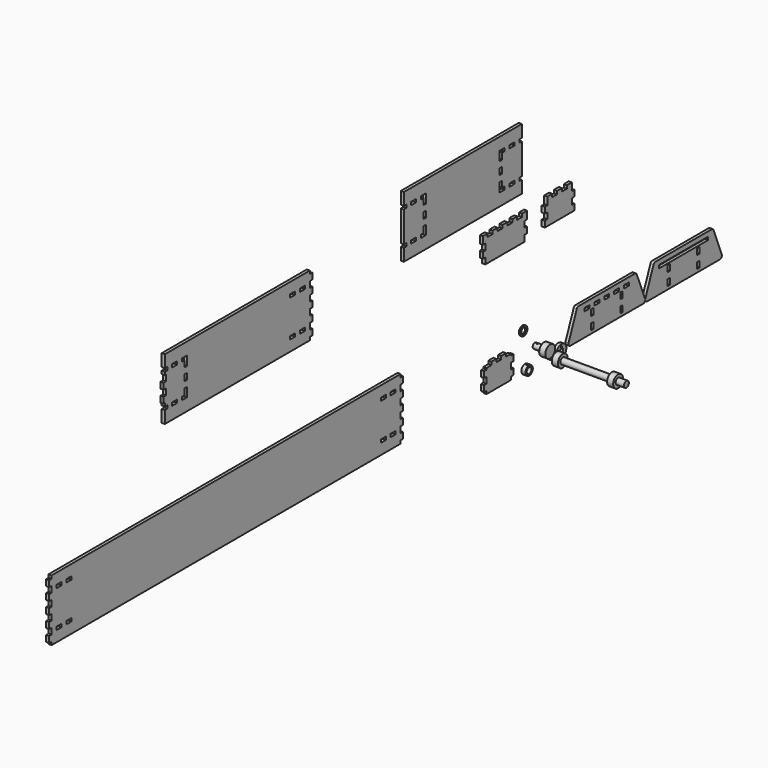
from build123d import *

# Parameters (mm, degrees)
F0_W      = 152.4
F0_H      = 101.6
F0_W_2    = 6.35
F0_H_2    = 12.7
F1_DEPTH  = 6.35
F2_W      = 152.4
F2_H      = 101.6
F2_W_2    = 6.35
F2_H_2    = 12.7
F2_W_3    = 127
F2_H_3    = 6.35
F3_DEPTH  = 6.35
F5_DEPTH  = 6.35
F6_W      = 12.7
F6_H      = 6.35
F7_DEPTH  = 6.35
F8_R      = 5.715
F9_DEPTH  = 19.05
F10_R     = 5.715
F11_DEPTH = 17.145
F12_R     = 12.7
F12_R_2   = 5.715
F13_DEPTH = 12.7
F14_R     = 6.35
F15_DEPTH = 101.6
F16_R     = 12.7
F16_R_2   = 6.35
F17_DEPTH = 12.7
F18_R     = 6.35
F19_DEPTH = 17.145
F20_R     = 12.7
F20_R_2   = 5.715
F21_DEPTH = 12.7
F22_R     = 1.5875
F23_DEPTH = 127.001
F24_R     = 9.525
F25_DEPTH = 8.4666666667
F26_R     = 1.5875
F27_DEPTH = 127.001
F28_R     = 6.35
F29_DEPTH = 8.4676667667
F30_R     = 9.525
F30_R_2   = 6.35
F31_DEPTH = 2.38125
F35_DEPTH = 6.35
F37_DEPTH = 6.35
F38_W     = 12.7
F38_H     = 6.35
F38_W_2   = 6.35
F38_H_2   = 12.7
F39_DEPTH = 6.35
F40_W     = 12.7
F40_H     = 6.35
F40_W_2   = 3.175
F40_H_2   = 12.7
F41_DEPTH = 6.35
F42_W     = 152.4
F42_H     = 38.1
F43_DEPTH = 6.35
F44_W     = 152.4
F44_H     = 38.1
F45_DEPTH = 6.35
F47_DEPTH = 6.35
F48_R     = 5.08
F50_DEPTH = 6.35
F51_R     = 5.08
F52_R     = 12.7
F52_R_2   = 1.524
F52_R_3   = 4.445
F53_DEPTH = 6.35


with BuildPart() as f1:
    # F0 (on Right) → F1 (new body)
    with BuildSketch(Plane.YZ):
        with Locations((76.2, 50.8)):
            Rectangle(F0_W, F0_H)
        with Locations((38.1, 12.7)):
            Rectangle(F0_W_2, F0_H_2, mode=Mode.SUBTRACT)
        with Locations((38.1, 38.1)):
            Rectangle(F0_W_2, F0_H_2, mode=Mode.SUBTRACT)
        Polygon((19.05, 53.975), (25.4, 53.975), (31.75, 53.975), (31.75, 50.8), (31.75, 47.625), (25.4, 47.625), (19.05, 47.625), (19.05, 50.8), align=None, mode=Mode.SUBTRACT)
        Polygon((44.45, 53.975), (50.8, 53.975), (57.15, 53.975), (57.15, 50.8), (57.15, 47.625), (50.8, 47.625), (44.45, 47.625), (44.45, 50.8), align=None, mode=Mode.SUBTRACT)
        Polygon((69.85, 53.975), (76.2, 53.975), (82.55, 53.975), (82.55, 50.8), (82.55, 47.625), (76.2, 47.625), (69.85, 47.625), (69.85, 50.8), align=None, mode=Mode.SUBTRACT)
        with Locations((114.3, 12.7)):
            Rectangle(F0_W_2, F0_H_2, mode=Mode.SUBTRACT)
        Polygon((95.25, 53.975), (101.6, 53.975), (107.95, 53.975), (107.95, 50.8), (107.95, 47.625), (101.6, 47.625), (95.25, 47.625), (95.25, 50.8), align=None, mode=Mode.SUBTRACT)
        with Locations((114.3, 38.1)):
            Rectangle(F0_W_2, F0_H_2, mode=Mode.SUBTRACT)
        Polygon((120.65, 53.975), (127, 53.975), (133.35, 53.975), (133.35, 50.8), (133.35, 47.625), (127, 47.625), (120.65, 47.625), (120.65, 50.8), align=None, mode=Mode.SUBTRACT)
    extrude(amount=F1_DEPTH)

    # F44 (on face) → F45 (cut, through all)
    with BuildSketch(Plane(origin=(0, 0, 0), x_dir=(0, -1, 0), z_dir=(-1, 0, 0))):
        with Locations((-76.2, 82.55)):
            Rectangle(F44_W, F44_H)
    extrude(amount=-F45_DEPTH, mode=Mode.SUBTRACT)

    # F49 (on face) → F50 (join)
    with BuildSketch(Plane(origin=(0, 0, 0), x_dir=(0, -1, 0), z_dir=(-1, 0, 0))):
        Polygon((-152.4, 0), (-152.4, 63.5), (-177.8, 0), align=None)
        Polygon((25.4, 0), (0, 63.5), (0, 0), align=None)
    extrude(amount=-F50_DEPTH)

    # F51
    f51_edges = [f1.edges().sort_by_distance(p)[0] for p in [
        (3.175, 152.4, 63.5),
        (3.175, 0, 63.5),
        (3.175, -25.4, 0),
        (3.175, 177.8, 0),
    ]]
    fillet(f51_edges, radius=F51_R)


with BuildPart() as f3:
    # F2 (on Right) → F3 (new body)
    with BuildSketch(Plane.YZ):
        with Locations((274.5815088749, 50.8)):
            Rectangle(F2_W, F2_H)
        with Locations((236.4815088749, 12.7)):
            Rectangle(F2_W_2, F2_H_2, mode=Mode.SUBTRACT)
        with Locations((236.4815088749, 38.1)):
            Rectangle(F2_W_2, F2_H_2, mode=Mode.SUBTRACT)
        with Locations((274.5815088749, 50.8)):
            Rectangle(F2_W_3, F2_H_3, mode=Mode.SUBTRACT)
        with Locations((312.6815088749, 12.7)):
            Rectangle(F2_W_2, F2_H_2, mode=Mode.SUBTRACT)
        with Locations((312.6815088749, 38.1)):
            Rectangle(F2_W_2, F2_H_2, mode=Mode.SUBTRACT)
    extrude(amount=F3_DEPTH)

    # F42 (on face) → F43 (cut, through all)
    with BuildSketch(Plane(origin=(0, 0, 0), x_dir=(0, -1, 0), z_dir=(-1, 0, 0))):
        with Locations((-274.5815088749, 82.55)):
            Rectangle(F42_W, F42_H)
    extrude(amount=-F43_DEPTH, mode=Mode.SUBTRACT)

    # F46 (on face) → F47 (join)
    with BuildSketch(Plane(origin=(0, 0, 0), x_dir=(0, -1, 0), z_dir=(-1, 0, 0))):
        Polygon((-350.7815088749, 0), (-350.7815088749, 63.5), (-376.1815088749, 0), align=None)
        Polygon((-172.9815088749, 0), (-198.3815088749, 63.5), (-198.3815088749, 0), align=None)
    extrude(amount=-F47_DEPTH)

    # F48
    f48_edges = [f3.edges().sort_by_distance(p)[0] for p in [
        (3.175, 350.781509, 63.5),
        (3.175, 198.381509, 63.5),
        (3.175, 376.181509, 0),
        (3.175, 172.981509, 0),
    ]]
    fillet(f48_edges, radius=F48_R)


with BuildPart() as f5:
    # F4 (on Right) → F5 (new body)
    with BuildSketch(Plane.YZ):
        Polygon((-234.6794404593, 0), (-171.1794404593, 0), (-171.1794404593, 6.35), (-164.8294404593, 6.35), (-164.8294404593, 19.05), (-171.1794404593, 19.05), (-171.1794404593, 31.75), (-164.8294404593, 31.75), (-164.8294404593, 44.45), (-171.1794404593, 44.45), (-171.1794404593, 47.625), (-183.8794404593, 47.625), (-183.8794404593, 53.975), (-196.5794404593, 53.975), (-196.5794404593, 47.625), (-202.9294404593, 47.625), (-209.2794404593, 47.625), (-209.2794404593, 53.975), (-221.9794404593, 53.975), (-221.9794404593, 47.625), (-234.6794404593, 47.625), (-234.6794404593, 44.45), (-241.0294404593, 44.45), (-241.0294404593, 31.75), (-234.6794404593, 31.75), (-234.6794404593, 19.05), (-241.0294404593, 19.05), (-241.0294404593, 6.35), (-234.6794404593, 6.35), align=None)
    extrude(amount=F5_DEPTH)


with BuildPart() as f7:
    # F6 (on Right) → F7 (new body)
    with BuildSketch(Plane.YZ):
        Polygon((-1358.3947817802, 0), (-456.6947817802, 0), (-456.6947817802, 6.35), (-450.3447817802, 6.35), (-450.3447817802, 19.05), (-456.6947817802, 19.05), (-456.6947817802, 22.225), (-456.6947817802, 28.575), (-456.6947817802, 31.75), (-450.3447817802, 31.75), (-450.3447817802, 44.45), (-456.6947817802, 44.45), (-456.6947817802, 57.15), (-450.3447817802, 57.15), (-450.3447817802, 69.85), (-456.6947817802, 69.85), (-456.6947817802, 82.55), (-450.3447817802, 82.55), (-450.3447817802, 95.25), (-456.6947817802, 95.25), (-456.6947817802, 98.425), (-456.6947817802, 104.775), (-456.6947817802, 107.95), (-450.3447817802, 107.95), (-450.3447817802, 120.65), (-456.6947817802, 120.65), (-456.6947817802, 127), (-1358.3947817802, 127), (-1358.3947817802, 120.65), (-1364.7447817802, 120.65), (-1364.7447817802, 107.95), (-1358.3947817802, 107.95), (-1358.3947817802, 104.775), (-1358.3947817802, 98.425), (-1358.3947817802, 95.25), (-1364.7447817802, 95.25), (-1364.7447817802, 82.55), (-1358.3947817802, 82.55), (-1358.3947817802, 69.85), (-1364.7447817802, 69.85), (-1364.7447817802, 57.15), (-1358.3947817802, 57.15), (-1358.3947817802, 44.45), (-1364.7447817802, 44.45), (-1364.7447817802, 31.75), (-1358.3947817802, 31.75), (-1358.3947817802, 28.575), (-1358.3947817802, 22.225), (-1358.3947817802, 19.05), (-1364.7447817802, 19.05), (-1364.7447817802, 6.35), (-1358.3947817802, 6.35), align=None)
        with Locations((-1339.3447817802, 25.4)):
            Rectangle(F6_W, F6_H, mode=Mode.SUBTRACT)
        with Locations((-1313.9447817802, 25.4)):
            Rectangle(F6_W, F6_H, mode=Mode.SUBTRACT)
        with Locations((-501.1447817802, 25.4)):
            Rectangle(F6_W, F6_H, mode=Mode.SUBTRACT)
        with Locations((-475.7447817802, 25.4)):
            Rectangle(F6_W, F6_H, mode=Mode.SUBTRACT)
        with Locations((-1339.3447817802, 101.6)):
            Rectangle(F6_W, F6_H, mode=Mode.SUBTRACT)
        with Locations((-1313.9447817802, 101.6)):
            Rectangle(F6_W, F6_H, mode=Mode.SUBTRACT)
        with Locations((-501.1447817802, 101.6)):
            Rectangle(F6_W, F6_H, mode=Mode.SUBTRACT)
        with Locations((-475.7447817802, 101.6)):
            Rectangle(F6_W, F6_H, mode=Mode.SUBTRACT)
    extrude(amount=F7_DEPTH)


with BuildPart() as f9:
    # F8 (on Right) → F9 (new body)
    with BuildSketch(Plane.YZ):
        with Locations((-101.6, 32.0885106921)):
            Circle(F8_R)
    extrude(amount=F9_DEPTH)

    # F20 (on face) → F21 (join)
    with BuildSketch(Plane.YZ.offset(19.05)):
        with Locations((-101.6, 32.0885106921)):
            Circle(F20_R)
        with Locations((-101.6, 32.0885106921)):
            Circle(F20_R_2, mode=Mode.SUBTRACT)
        with Locations((-101.6, 32.0885106921)):
            Circle(F20_R_2)
    extrude(amount=F21_DEPTH)

    # F22 (on Top) → F23 (cut, through all)
    with BuildSketch(Plane.XY):
        with Locations((4.7625, -101.6)):
            Circle(F22_R)
    extrude(amount=F23_DEPTH, mode=Mode.SUBTRACT)


with BuildPart() as f11:
    # F10 (on Right) → F11 (new body)
    with BuildSketch(Plane.YZ):
        with Locations((-66.7278746938, 0)):
            Circle(F10_R)
    extrude(amount=F11_DEPTH)

    # F12 (on face) → F13 (join)
    with BuildSketch(Plane.YZ.offset(17.145)):
        with Locations((-66.7278746938, 0)):
            Circle(F12_R)
        with Locations((-66.7278746938, 0)):
            Circle(F12_R_2, mode=Mode.SUBTRACT)
        with Locations((-66.7278746938, 0)):
            Circle(F12_R_2)
    extrude(amount=F13_DEPTH)

    # F14 (on face) → F15 (join)
    with BuildSketch(Plane.YZ.offset(29.845)):
        with Locations((-66.7278746938, 0)):
            Circle(F14_R)
    extrude(amount=F15_DEPTH)

    # F16 (on face) → F17 (join)
    with BuildSketch(Plane.YZ.offset(131.445)):
        with Locations((-66.7278746938, 0)):
            Circle(F16_R)
        with Locations((-66.7278746938, 0)):
            Circle(F16_R_2, mode=Mode.SUBTRACT)
        with Locations((-66.7278746938, 0)):
            Circle(F16_R_2)
    extrude(amount=F17_DEPTH)

    # F18 (on face) → F19 (join)
    with BuildSketch(Plane.YZ.offset(144.145)):
        with Locations((-66.7278746938, 0)):
            Circle(F18_R)
    extrude(amount=F19_DEPTH)


with BuildPart() as f25:
    # F24 (on Right) → F25 (new body)
    with BuildSketch(Plane.YZ):
        with Locations((-127, 0)):
            Circle(F24_R)
    extrude(amount=F25_DEPTH)

    # F26 (on Top) → F27 (cut, through all)
    with BuildSketch(Plane.XY):
        with Locations((4.2333333333, -127)):
            Circle(F26_R)
    extrude(amount=F27_DEPTH, mode=Mode.SUBTRACT)

    # F28 (on face) → F29 (cut, through all)
    with BuildSketch(Plane(origin=(0, 0, 0), x_dir=(0, -1, 0), z_dir=(-1, 0, 0))):
        with Locations((127, 0)):
            Circle(F28_R)
    extrude(amount=-F29_DEPTH, mode=Mode.SUBTRACT)


with BuildPart() as f31:
    # F30 (on Right) → F31 (new body)
    with BuildSketch(Plane.YZ):
        with Locations((-133.449241519, 72.6503282785)):
            Circle(F30_R)
        with Locations((-133.449241519, 72.6503282785)):
            Circle(F30_R_2, mode=Mode.SUBTRACT)
    extrude(amount=F31_DEPTH)


with BuildPart() as f32_1:
    # F32: copy of F5
    add(f5.part)


with BuildPart() as f35:
    # F34 (on Right) → F35 (new body)
    with BuildSketch(Plane.YZ):
        Polygon((-237.713524918, 249.9757648349), (-237.713524918, 237.2757648349), (-136.113524918, 237.2757648349), (-136.113524918, 249.9757648349), (-129.763524918, 249.9757648349), (-129.763524918, 262.6757648349), (-136.113524918, 262.6757648349), (-136.113524918, 275.3757648349), (-129.763524918, 275.3757648349), (-129.763524918, 291.2507648349), (-142.463524918, 291.2507648349), (-142.463524918, 284.9007648349), (-155.163524918, 284.9007648349), (-155.163524918, 291.2507648349), (-167.863524918, 291.2507648349), (-167.863524918, 284.9007648349), (-180.563524918, 284.9007648349), (-180.563524918, 291.2507648349), (-193.263524918, 291.2507648349), (-193.263524918, 284.9007648349), (-205.963524918, 284.9007648349), (-205.963524918, 291.2507648349), (-218.663524918, 291.2507648349), (-218.663524918, 284.9007648349), (-231.363524918, 284.9007648349), (-231.363524918, 291.2507648349), (-244.063524918, 291.2507648349), (-244.063524918, 275.3757648349), (-237.713524918, 275.3757648349), (-237.713524918, 262.6757648349), (-244.063524918, 262.6757648349), (-244.063524918, 249.9757648349), align=None)
    extrude(amount=F35_DEPTH)


with BuildPart() as f37:
    # F36 (on Right) → F37 (new body)
    with BuildSketch(Plane.YZ):
        Polygon((-83.9351456323, 254.5199484468), (-83.9351456323, 241.8199484468), (-7.7351456323, 241.8199484468), (-7.7351456323, 254.5199484468), (-14.0851456323, 254.5199484468), (-14.0851456323, 267.2199484468), (-7.7351456323, 267.2199484468), (-7.7351456323, 279.9199484468), (-14.0851456323, 279.9199484468), (-14.0851456323, 295.7949484468), (-26.7851456323, 295.7949484468), (-26.7851456323, 289.4449484468), (-39.4851456323, 289.4449484468), (-39.4851456323, 295.7949484468), (-52.1851456323, 295.7949484468), (-52.1851456323, 289.4449484468), (-64.8851456323, 289.4449484468), (-64.8851456323, 295.7949484468), (-77.5851456323, 295.7949484468), (-77.5851456323, 279.9199484468), (-83.9351456323, 279.9199484468), (-83.9351456323, 267.2199484468), (-77.5851456323, 267.2199484468), (-77.5851456323, 254.5199484468), align=None)
    extrude(amount=F37_DEPTH)


with BuildPart() as f39:
    # F38 (on Right) → F39 (new body)
    with BuildSketch(Plane.YZ):
        Polygon((-441.788833046, 353.0291121978), (-448.138833046, 353.0291121978), (-448.138833046, 327.6291121978), (-143.338833046, 327.6291121978), (-143.338833046, 353.0291121978), (-149.688833046, 353.0291121978), (-149.688833046, 359.3791121978), (-143.338833046, 359.3791121978), (-143.338833046, 422.8791121978), (-149.688833046, 422.8791121978), (-149.688833046, 429.2291121978), (-143.338833046, 429.2291121978), (-143.338833046, 454.6291121978), (-448.138833046, 454.6291121978), (-448.138833046, 429.2291121978), (-441.788833046, 429.2291121978), (-429.088833046, 429.2291121978), (-416.388833046, 429.2291121978), (-403.688833046, 429.2291121978), (-390.988833046, 429.2291121978), (-390.988833046, 422.8791121978), (-390.988833046, 410.1791121978), (-390.988833046, 397.4791121978), (-390.988833046, 384.7791121978), (-390.988833046, 372.0791121978), (-390.988833046, 359.3791121978), (-390.988833046, 353.0291121978), (-403.688833046, 353.0291121978), (-416.388833046, 353.0291121978), (-429.088833046, 353.0291121978), align=None)
        with Locations((-168.738833046, 356.2041121978)):
            Rectangle(F38_W, F38_H, mode=Mode.SUBTRACT)
        Polygon((-187.788833046, 359.3791121978), (-187.788833046, 353.0291121978), (-200.488833046, 353.0291121978), (-200.488833046, 359.3791121978), (-200.488833046, 372.0791121978), (-194.138833046, 372.0791121978), (-194.138833046, 359.3791121978), align=None, mode=Mode.SUBTRACT)
        with Locations((-197.313833046, 391.1291121978)):
            Rectangle(F38_W_2, F38_H_2, mode=Mode.SUBTRACT)
        Polygon((-194.138833046, 410.1791121978), (-200.488833046, 410.1791121978), (-200.488833046, 422.8791121978), (-200.488833046, 429.2291121978), (-187.788833046, 429.2291121978), (-187.788833046, 422.8791121978), (-194.138833046, 422.8791121978), align=None, mode=Mode.SUBTRACT)
        with Locations((-168.738833046, 426.0541121978)):
            Rectangle(F38_W, F38_H, mode=Mode.SUBTRACT)
        Polygon((-441.788833046, 359.3791121978), (-441.788833046, 353.0291121978), (-429.088833046, 353.0291121978), (-429.088833046, 359.3791121978), (-416.388833046, 359.3791121978), (-416.388833046, 353.0291121978), (-403.688833046, 353.0291121978), (-403.688833046, 359.3791121978), (-397.338833046, 359.3791121978), (-397.338833046, 372.0791121978), (-390.988833046, 372.0791121978), (-390.988833046, 384.7791121978), (-397.338833046, 384.7791121978), (-397.338833046, 397.4791121978), (-390.988833046, 397.4791121978), (-390.988833046, 410.1791121978), (-397.338833046, 410.1791121978), (-397.338833046, 422.8791121978), (-403.688833046, 422.8791121978), (-403.688833046, 429.2291121978), (-416.388833046, 429.2291121978), (-416.388833046, 422.8791121978), (-429.088833046, 422.8791121978), (-429.088833046, 429.2291121978), (-441.788833046, 429.2291121978), (-441.788833046, 422.8791121978), (-448.138833046, 422.8791121978), (-448.138833046, 359.3791121978), align=None)
    extrude(amount=F39_DEPTH)


with BuildPart() as f41:
    # F40 (on Right) → F41 (new body)
    with BuildSketch(Plane.YZ):
        Polygon((-691.2080654318, 289.8443043449), (-684.8580654318, 289.8443043449), (-684.8580654318, 302.5443043449), (-691.2080654318, 302.5443043449), (-691.2080654318, 305.7193043449), (-691.2080654318, 312.0693043449), (-691.2080654318, 315.2443043449), (-684.8580654318, 315.2443043449), (-684.8580654318, 327.9443043449), (-691.2080654318, 327.9443043449), (-691.2080654318, 340.6443043449), (-684.8580654318, 340.6443043449), (-684.8580654318, 353.3443043449), (-691.2080654318, 353.3443043449), (-691.2080654318, 366.0443043449), (-684.8580654318, 366.0443043449), (-684.8580654318, 378.7443043449), (-691.2080654318, 378.7443043449), (-691.2080654318, 381.9193043449), (-691.2080654318, 388.2693043449), (-691.2080654318, 391.4443043449), (-684.8580654318, 391.4443043449), (-684.8580654318, 404.1443043449), (-691.2080654318, 404.1443043449), (-691.2080654318, 410.4943043449), (-1065.8580654318, 410.4943043449), (-1065.8580654318, 385.0943043449), (-1062.6830654318, 385.0943043449), (-1059.5080654318, 385.0943043449), (-1046.8080654318, 385.0943043449), (-1034.1080654318, 385.0943043449), (-1021.4080654318, 385.0943043449), (-1015.0580654318, 385.0943043449), (-1008.7080654318, 385.0943043449), (-1008.7080654318, 378.7443043449), (-1008.7080654318, 366.0443043449), (-1008.7080654318, 353.3443043449), (-1008.7080654318, 340.6443043449), (-1008.7080654318, 327.9443043449), (-1008.7080654318, 315.2443043449), (-1008.7080654318, 308.8943043449), (-1015.0580654318, 308.8943043449), (-1021.4080654318, 308.8943043449), (-1034.1080654318, 308.8943043449), (-1046.8080654318, 308.8943043449), (-1059.5080654318, 308.8943043449), (-1062.6830654318, 308.8943043449), (-1065.8580654318, 308.8943043449), (-1065.8580654318, 283.4943043449), (-691.2080654318, 283.4943043449), align=None)
        with Locations((-735.6580654318, 308.8943043449)):
            Rectangle(F40_W, F40_H, mode=Mode.SUBTRACT)
        with Locations((-710.2580654318, 308.8943043449)):
            Rectangle(F40_W, F40_H, mode=Mode.SUBTRACT)
        with Locations((-735.6580654318, 385.0943043449)):
            Rectangle(F40_W, F40_H, mode=Mode.SUBTRACT)
        with Locations((-710.2580654318, 385.0943043449)):
            Rectangle(F40_W, F40_H, mode=Mode.SUBTRACT)
        Polygon((-1062.6830654318, 321.5943043449), (-1062.6830654318, 315.2443043449), (-1059.5080654318, 315.2443043449), (-1059.5080654318, 308.8943043449), (-1046.8080654318, 308.8943043449), (-1046.8080654318, 315.2443043449), (-1034.1080654318, 315.2443043449), (-1034.1080654318, 308.8943043449), (-1021.4080654318, 308.8943043449), (-1021.4080654318, 315.2443043449), (-1015.0580654318, 315.2443043449), (-1015.0580654318, 327.9443043449), (-1008.7080654318, 327.9443043449), (-1008.7080654318, 340.6443043449), (-1015.0580654318, 340.6443043449), (-1015.0580654318, 353.3443043449), (-1008.7080654318, 353.3443043449), (-1008.7080654318, 366.0443043449), (-1015.0580654318, 366.0443043449), (-1015.0580654318, 378.7443043449), (-1021.4080654318, 378.7443043449), (-1021.4080654318, 385.0943043449), (-1034.1080654318, 385.0943043449), (-1034.1080654318, 378.7443043449), (-1046.8080654318, 378.7443043449), (-1046.8080654318, 385.0943043449), (-1059.5080654318, 385.0943043449), (-1059.5080654318, 378.7443043449), (-1062.6830654318, 378.7443043449), (-1062.6830654318, 372.3943043449), (-1062.6830654318, 359.6943043449), (-1062.6830654318, 346.9943043449), (-1062.6830654318, 334.2943043449), align=None)
        with Locations((-1064.2705654318, 353.3443043449)):
            Rectangle(F40_W_2, F40_H_2)
        with Locations((-1067.4455654318, 353.3443043449)):
            Rectangle(F40_W_2, F40_H_2)
        with Locations((-1064.2705654318, 327.9443043449)):
            Rectangle(F40_W_2, F40_H_2)
        with Locations((-1067.4455654318, 327.9443043449)):
            Rectangle(F40_W_2, F40_H_2)
        with Locations((-1064.2705654318, 318.4193043449)):
            Rectangle(F40_W_2, F40_H)
        with Locations((-1064.2705654318, 375.5693043449)):
            Rectangle(F40_W_2, F40_H)
    extrude(amount=F41_DEPTH)


with BuildPart() as f53:
    # F52 (on Right) → F53 (new body)
    with BuildSketch(Plane.YZ):
        with Locations((-40.9202546468, 0)):
            Circle(F52_R)
        with Locations((-40.9202546468, -7.3025)):
            Circle(F52_R_2, mode=Mode.SUBTRACT)
        with Locations((-40.9202546468, 0)):
            Circle(F52_R_3, mode=Mode.SUBTRACT)
        with Locations((-40.9202546468, 7.3025)):
            Circle(F52_R_2, mode=Mode.SUBTRACT)
    extrude(amount=F53_DEPTH)


solid = Compound([f1.part, f3.part, f5.part, f7.part, f9.part, f11.part, f25.part, f31.part, f35.part, f37.part, f39.part, f41.part, f53.part])
